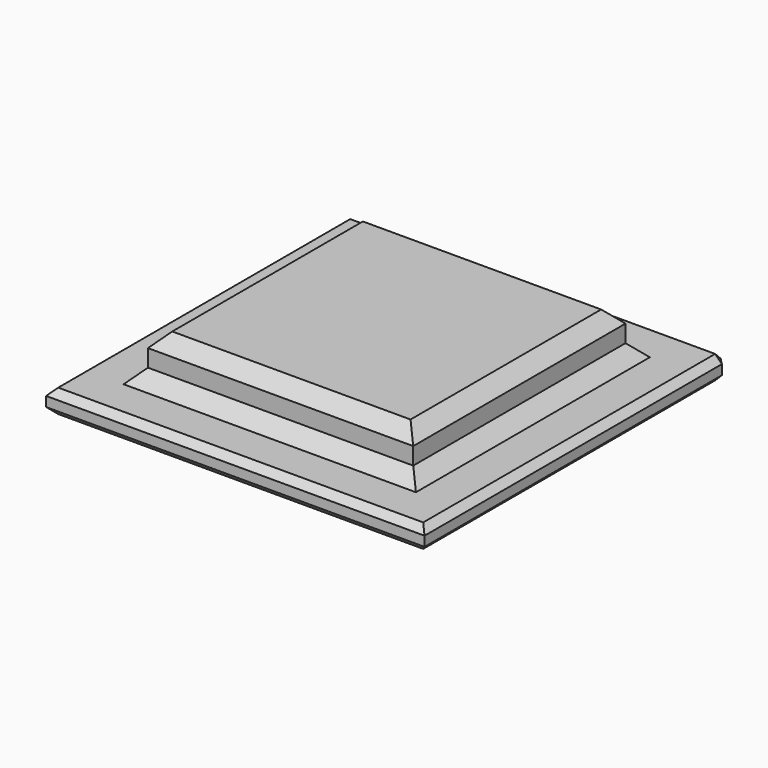
from build123d import *

# Parameters (mm, degrees)
F0_W     = 142.24
F0_H     = 142.24
F1_DEPTH = 8.763
F2_W     = 99.7141572639
F2_H     = 99.7141572639
F3_DEPTH = 25.4
F4_SIZE  = 2.54
F5_SIZE  = 5.08


with BuildPart() as f1:
    # F0 (on Top) → F1 (new body)
    with BuildSketch(Plane.XY):
        Rectangle(F0_W, F0_H)
    extrude(amount=F1_DEPTH)

    # F2 (on Top) → F3 (join)
    with BuildSketch(Plane.XY):
        Rectangle(F2_W, F2_H)
    extrude(amount=F3_DEPTH)

    # F4
    f4_edges = [f1.edges().sort_by_distance(p)[0] for p in [
        (71.12, 71.12, 4.3815),
        (-71.12, 71.12, 4.3815),
        (0, 71.12, 0),
        (0, 71.12, 8.763),
        (71.12, 0, 8.763),
        (71.12, 0, 0),
        (0, -71.12, 8.763),
        (0, -71.12, 0),
        (-71.12, 0, 8.763),
        (-71.12, 0, 0),
    ]]
    chamfer(f4_edges, length=F4_SIZE)

    # F5
    f5_edges = [f1.edges().sort_by_distance(p)[0] for p in [
        (-49.857079, 0, 25.4),
        (0, 49.857079, 25.4),
        (0, -49.857079, 25.4),
        (49.857079, 0, 25.4),
        (-49.857079, 0, 8.763),
        (0, 49.857079, 8.763),
        (49.857079, 0, 8.763),
        (0, -49.857079, 8.763),
    ]]
    chamfer(f5_edges, length=F5_SIZE)


solid = f1.part
